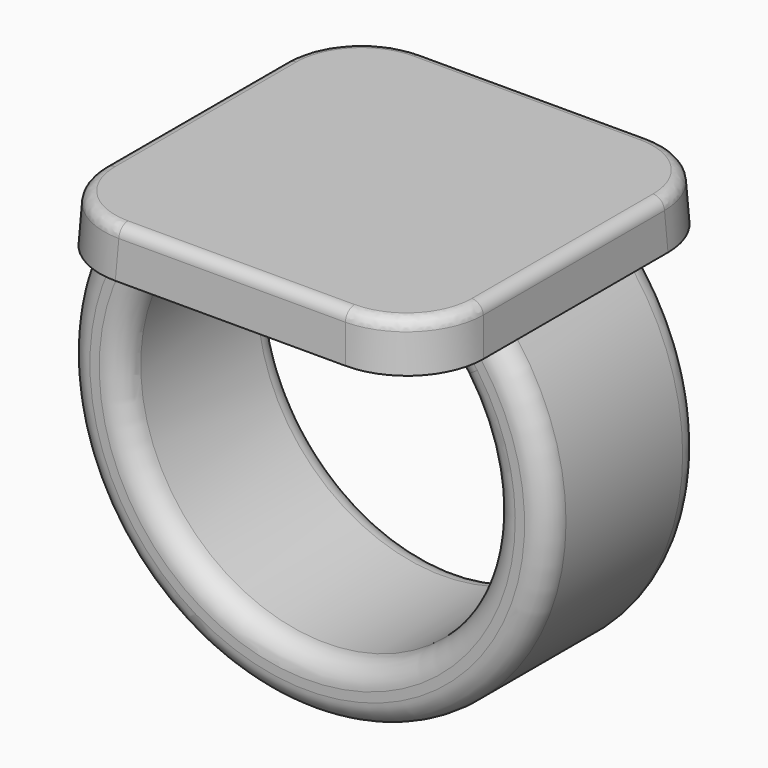
from build123d import *

# Parameters (mm, degrees)
F0_W          = 25.4
F0_H          = 25.4
F1_DEPTH      = 3.175
F1_TAPER      = 3
F3_W          = 5.08
F3_H          = 12.7
F6_DEPTH      = 6.35
F6_DEPTH_BACK = 6.35
F7_R          = 5.08
F8_R          = 1.524
F9_R          = 0.762


with BuildPart() as f1:
    # F0 (on Top) → F1 (new body)
    with BuildSketch(Plane.XY):
        Rectangle(F0_W, F0_H)
    extrude(amount=F1_DEPTH, taper=F1_TAPER)

    # F4: sweep along a path in F2
    with BuildLine(Plane.XZ) as f4_path:
        ThreePointArc((-10.16, 0), (0, -23.5582897328), (10.16, 0))
    # F3 (on face) → F4 (sweep)
    with BuildSketch(Plane(origin=(0, 0, 0), x_dir=(1, 0, 0), z_dir=(0, 0, -1))):
        with Locations((-10.16, 0)):
            Rectangle(F3_W, F3_H)
    sweep(path=f4_path.line)

    # F5 (on Front) → F6 (join, two sides)
    with BuildSketch(Plane.XZ) as f6_sk:
        with BuildLine():
            Line((10.0130578512, -2.535746045), (10.16, 0))
            Line((10.16, 0), (7.62, 0))
            ThreePointArc((7.62, 0), (8.9072265211, -1.1822790439), (10.0130578512, -2.535746045))
        make_face()
    extrude(amount=F6_DEPTH)
    extrude(f6_sk.sketch, amount=-F6_DEPTH_BACK)

    # F7
    f7_edges = [f1.edges().sort_by_distance(p)[0] for p in [
        (-12.616803, 12.616803, 1.5875),
        (12.616803, 12.616803, 1.5875),
        (12.616803, -12.616803, 1.5875),
        (-12.616803, -12.616803, 1.5875),
    ]]
    fillet(f7_edges, radius=F7_R)

    # F8
    f8_edges = [f1.edges().sort_by_distance(p)[0] for p in [
        (-1.743325, -6.35, -21.711017),
        (8.907227, -6.35, -1.182279),
        (-1.743325, 6.35, -21.711017),
        (0, -6.35, -25.501344),
        (0, 6.35, -25.501344),
        (8.907227, 6.35, -1.182279),
    ]]
    fillet(f8_edges, radius=F8_R)

    # F9
    f9_edges = [f1.edges().sort_by_distance(p)[0] for p in [
        (0, -12.533605, 3.175),
        (-11.048589, -11.048589, 3.175),
        (11.048589, -11.048589, 3.175),
        (-12.533605, 0, 3.175),
        (12.533605, 0, 3.175),
        (-11.048589, 11.048589, 3.175),
        (11.048589, 11.048589, 3.175),
        (0, 12.533605, 3.175),
    ]]
    fillet(f9_edges, radius=F9_R)


solid = f1.part
